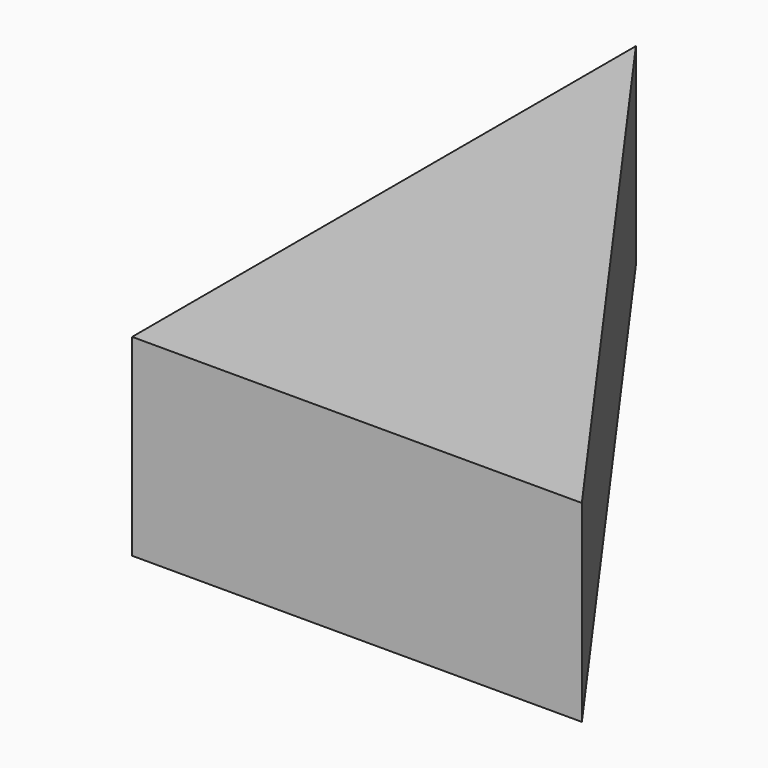
from build123d import *

# Parameters (mm, degrees)
F0_W        = 14
F0_H        = 6
F1_DEPTH    = 20
F2_T1_DEPTH = 109.2812557381


# Not quite as in the source:
# - a fillet or chamfer that OpenCascade refuses, or shapes differently, is made with other operations: its cross-section is extruded or revolved along the edge and cut away or added


with BuildPart() as f1:
    # F0 (on Front) → F1 (new body)
    with BuildSketch(Plane.XZ):
        Rectangle(F0_W, F0_H)
    extrude(amount=F1_DEPTH)

    # F2: chamfer of 14.2837 x 20 on 1 edges, made by hand

    # F2_s2 → F2_t1 (cut)
    with BuildSketch(Plane.XY.offset(-54.640627869)):
        Polygon((7, -20), (-7.2837, 0), (7, 0), align=None)
    extrude(amount=F2_T1_DEPTH, mode=Mode.SUBTRACT)


solid = f1.part
